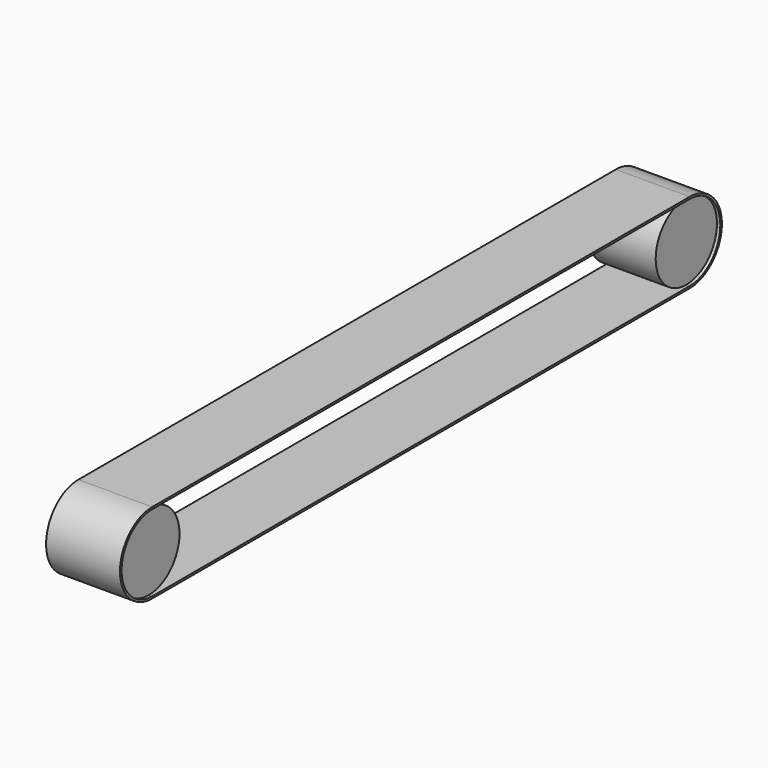
from build123d import *

# Parameters (mm, degrees)
F1_DEPTH = 100
F2_DEPTH = 105
F3_DEPTH = 5


with BuildPart() as f1:
    # F0 (on Right) → F1 (new body)
    with BuildSketch(Plane.YZ):
        with BuildLine():
            ThreePointArc((-943, 0), (-959.6949134724, 40.3050865276), (-1000, 57))
            ThreePointArc((-1000, 57), (-1057, 0), (-1000, -57))
            ThreePointArc((-1000, -57), (-959.6949134724, -40.3050865276), (-943, 0))
        make_face()
    extrude(amount=F1_DEPTH)


with BuildPart() as f1b:
    # F0 (on Right) → F1, piece 2 (new body)
    with BuildSketch(Plane.YZ):
        with BuildLine():
            ThreePointArc((57, 0), (40.3050865276, 40.3050865276), (0, 57))
            ThreePointArc((0, 57), (-57, 0), (0, -57))
            ThreePointArc((0, -57), (40.3050865276, -40.3050865276), (57, 0))
        make_face()
    extrude(amount=F1_DEPTH)


with BuildPart() as f2:
    # F0 (on Right) → F2 (new body)
    with BuildSketch(Plane.YZ):
        with BuildLine():
            Line((-1000, -60), (0, -60))
            ThreePointArc((0, -60), (60, 0), (0, 60))
            Line((0, 60), (-1000, 60))
            ThreePointArc((-1000, 60), (-1060, 0), (-1000, -60))
        make_face()
        with BuildLine():
            ThreePointArc((-1000, -57), (-1057, 0), (-1000, 57))
            Line((-1000, 57), (0, 57))
            ThreePointArc((0, 57), (40.3050865276, 40.3050865276), (57, 0))
            ThreePointArc((57, 0), (40.3050865276, -40.3050865276), (0, -57))
            Line((0, -57), (-1000, -57))
        make_face(mode=Mode.SUBTRACT)
    extrude(amount=F2_DEPTH)

    # F0 (on Right) → F3 (join)
    with BuildSketch(Plane.YZ):
        with BuildLine():
            Line((-1000, -60), (0, -60))
            ThreePointArc((0, -60), (60, 0), (0, 60))
            Line((0, 60), (-1000, 60))
            ThreePointArc((-1000, 60), (-1060, 0), (-1000, -60))
        make_face()
        with BuildLine():
            ThreePointArc((-1000, -57), (-1057, 0), (-1000, 57))
            Line((-1000, 57), (0, 57))
            ThreePointArc((0, 57), (40.3050865276, 40.3050865276), (57, 0))
            ThreePointArc((57, 0), (40.3050865276, -40.3050865276), (0, -57))
            Line((0, -57), (-1000, -57))
        make_face(mode=Mode.SUBTRACT)
    extrude(amount=-F3_DEPTH)


solid = Compound([f1.part, f1b.part, f2.part])
